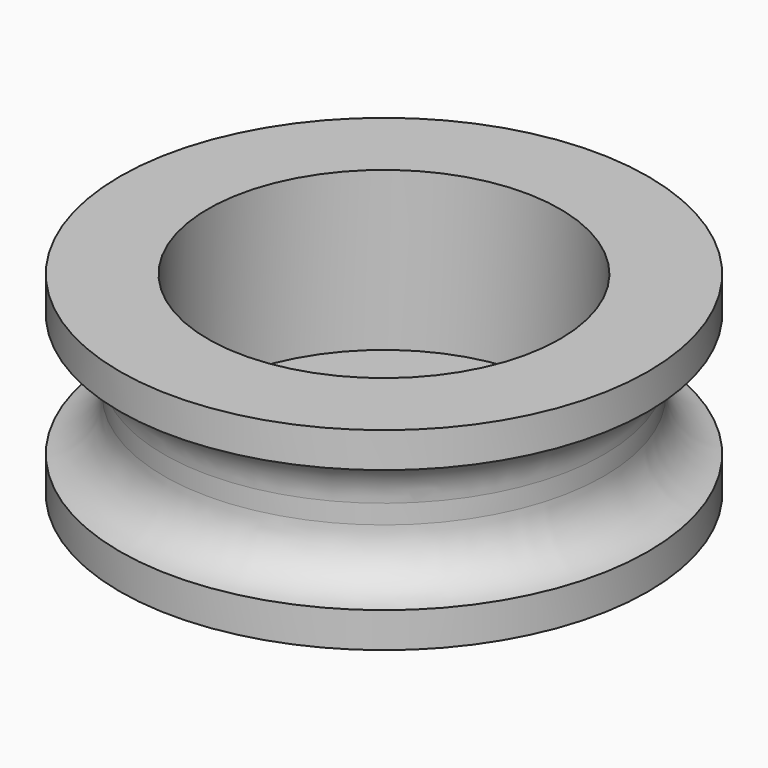
from build123d import *

# Parameters (mm, degrees)
F0_R     = 15
F0_R_2   = 12.5
F0_R_3   = 10
F0_R_4   = 7
F1_DEPTH = 2
F2_DEPTH = 9
F3_R     = 15
F3_R_2   = 12.5
F3_R_3   = 10
F4_DEPTH = 2


# Not quite as in the source:
# - a fillet or chamfer that OpenCascade refuses, or shapes differently, is made with other operations: its cross-section is extruded or revolved along the edge and cut away or added


with BuildPart() as f1:
    # F0 (on Top) → F1 (new body)
    with BuildSketch(Plane.XY):
        Circle(F0_R)
        Circle(F0_R_2, mode=Mode.SUBTRACT)
        Circle(F0_R_2)
        Circle(F0_R_3, mode=Mode.SUBTRACT)
        Circle(F0_R_3)
        Circle(F0_R_4, mode=Mode.SUBTRACT)
    extrude(amount=F1_DEPTH)

    # F0 (on Top) → F2 (join)
    with BuildSketch(Plane.XY):
        Circle(F0_R_2)
        Circle(F0_R_3, mode=Mode.SUBTRACT)
    extrude(amount=F2_DEPTH)

    # F3 (on face) → F4 (join)
    with BuildSketch(Plane.XY.offset(9)):
        Circle(F3_R)
        Circle(F3_R_2, mode=Mode.SUBTRACT)
        Circle(F3_R_2)
        Circle(F3_R_3, mode=Mode.SUBTRACT)
    extrude(amount=F4_DEPTH)

    # F5: fillet of radius 3 on 2 edges, made by hand

    # F5_s1 → F5_t2 (revolve)
    with BuildSketch(Plane.XZ):
        with BuildLine():
            ThreePointArc((12.5, 4.9580398916), (13.2087121525, 3.0215482184), (15, 2))
            Line((15, 2), (12.5, 2))
            Line((12.5, 2), (12.5, 4.9580398916))
        make_face()
    revolve(axis=Axis((0, 0, 2), (0, 0, -1)))

    # F5_s3 → F5_t4 (revolve)
    with BuildSketch(Plane.XZ):
        with BuildLine():
            ThreePointArc((15, 9), (13.2087121525, 7.9784517816), (12.5, 6.0419601084))
            Line((12.5, 6.0419601084), (12.5, 9))
            Line((12.5, 9), (15, 9))
        make_face()
    revolve(axis=Axis((0, 0, 9), (0, 0, 1)))


solid = f1.part
